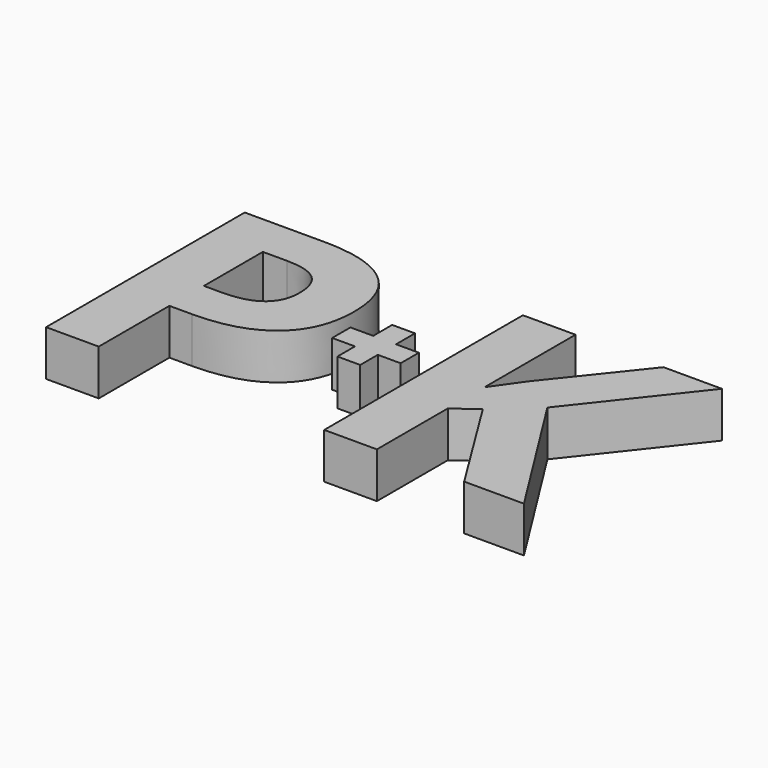
from build123d import *

# Parameters (mm, degrees)
F0_W         = 2.538538454
F0_H         = 2.54
F0_W_2       = 2.54
F0_H_2       = 2.6371062424
F0_W_3       = 2.541461546
F0_H_3       = 2.4428937576
F1_DEPTH     = 5.08
F2_TEXT_SIZE = 38.7208859643
F3_DEPTH     = 5.08


# Not quite as in the source:
# - Text() gives the source's letters only with a copy of the font that has no kerning and outlines rounded to 1/6400 em; it was checked with that copy


with BuildPart() as f1:
    # F0 (on Top) → F1 (new body)
    with BuildSketch(Plane.XY):
        with Locations((-2.5404215096, -0.0128386389)):
            Rectangle(F0_W, F0_H)
        with Locations((-0.0011522826, -0.0128386389)):
            Rectangle(F0_W_2, F0_H)
        with Locations((-0.0011522826, 2.5757144823)):
            Rectangle(F0_W_2, F0_H_2)
        with Locations((2.5395784904, -0.0128386389)):
            Rectangle(F0_W_3, F0_H)
        with Locations((-0.0011522826, -2.5042855177)):
            Rectangle(F0_W_2, F0_H_3)
    extrude(amount=F1_DEPTH)


with BuildPart() as f3:
    # F2 (on Top) → F3 (new body)
    with BuildSketch(Plane.XY):
        with Locations((-27.9809143394, -15.2310701087)):
            Text('P', F2_TEXT_SIZE, font='Open Sans', font_style=FontStyle.BOLD, text_align=(TextAlign.LEFT, TextAlign.BOTTOM))
        with Locations((2.9852187727, -15.2310701087)):
            Text('K', F2_TEXT_SIZE, font='Open Sans', font_style=FontStyle.BOLD, text_align=(TextAlign.LEFT, TextAlign.BOTTOM))
    extrude(amount=F3_DEPTH)


solid = Compound([f1.part, f3.part])
